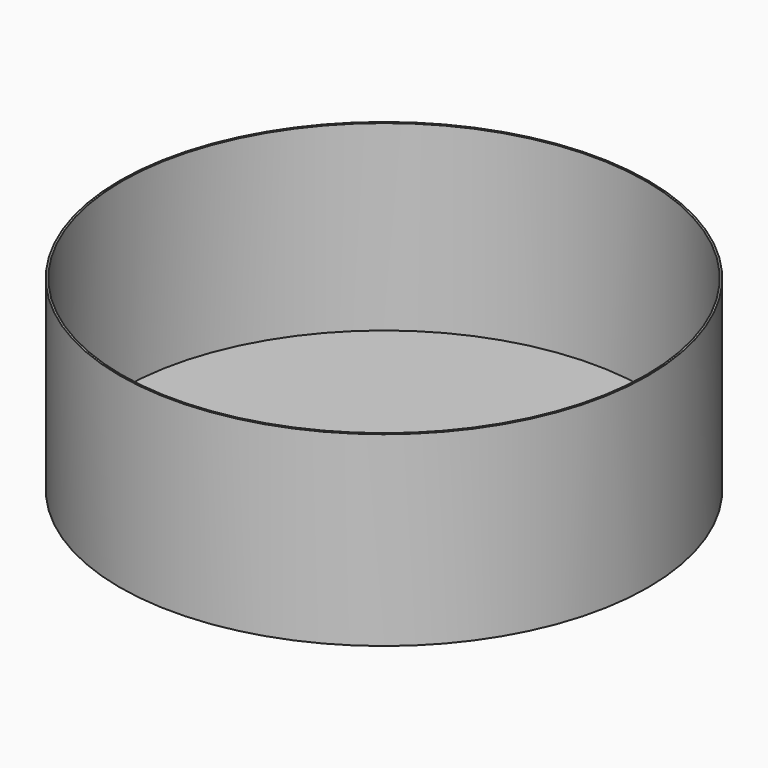
from build123d import *

# Parameters (mm, degrees)
F0_R     = 107.95
F0_R_2   = 107.15625
F1_DEPTH = 76.2
F2_DEPTH = 1.5875


# Not quite as in the source:
# - a length typed as a fraction of an inch, garbled in the dataset ("3 / 203.2 mm" for 3/8 in), is restored


with BuildPart() as f1:
    # F0 (on Top) → F1 (new body)
    with BuildSketch(Plane.XY):
        Circle(F0_R)
        Circle(F0_R_2, mode=Mode.SUBTRACT)
    extrude(amount=F1_DEPTH)

    # F0 (on Top) → F2 (join)
    with BuildSketch(Plane.XY):
        Circle(F0_R_2)
    extrude(amount=F2_DEPTH)


solid = f1.part
